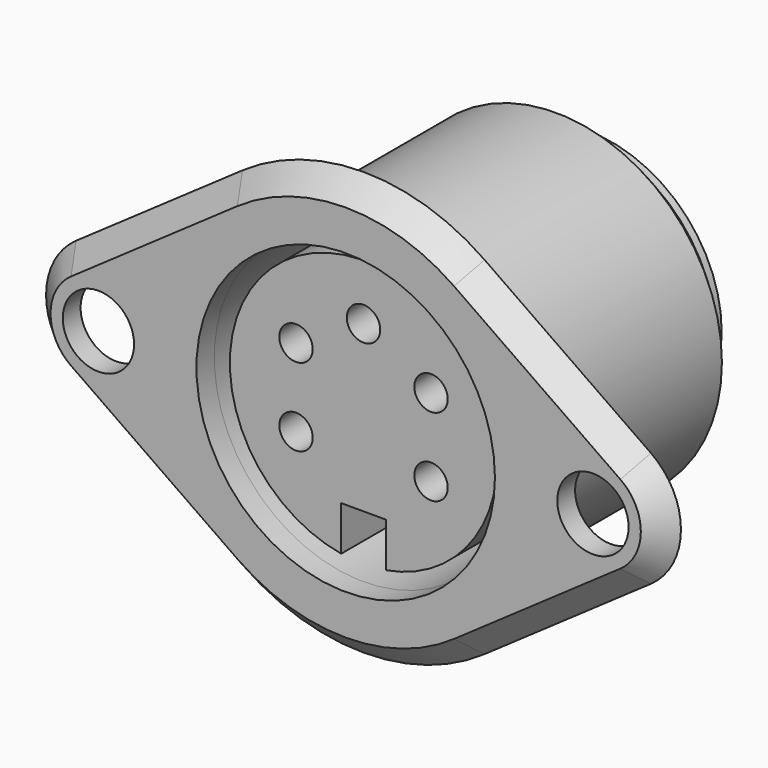
from build123d import *

# Parameters (mm, degrees)
F0_R     = 1.6
F0_R_2   = 7.45
F0_R_3   = 6.7
F1_DEPTH = 1
F2_SIZE  = 0.99999
F0_R_4   = 0.75
F3_DEPTH = 12.1
F4_T     = 0.75
F5_DEPTH = 12.6
F6_DEPTH = 10
F7_SIZE  = 1.3


# Not quite as in the source:
# - a fillet or chamfer is up to 0.001 mm smaller than in the source, because OpenCascade refuses the exact size
# - a shell that OpenCascade refuses in one call is made with other operations: the cavity is built on its own and cut out
# - a feature names something its author has since deleted; it is built from what else it names


with BuildPart() as f1:
    # F0 (on Front) → F1 (new body)
    with BuildSketch(Plane.XZ):
        with BuildLine():
            Line((-5.4346846847, 7.7919318771), (-12.902027027, 2.5836405698))
            ThreePointArc((-12.902027027, 2.5836405698), (-14.25, 0), (-12.902027027, -2.5836405698))
            Line((-12.902027027, -2.5836405698), (-5.4346846847, -7.7919318771))
            ThreePointArc((-5.4346846847, -7.7919318771), (0, -9.5), (5.4346846847, -7.7919318771))
            Line((5.4346846847, -7.7919318771), (12.902027027, -2.5836405698))
            ThreePointArc((12.902027027, -2.5836405698), (14.25, 0), (12.902027027, 2.5836405698))
            Line((12.902027027, 2.5836405698), (5.4346846847, 7.7919318771))
            ThreePointArc((5.4346846847, 7.7919318771), (0, 9.5), (-5.4346846847, 7.7919318771))
        make_face()
        with Locations((-11.1, 0)):
            Circle(F0_R, mode=Mode.SUBTRACT)
        Circle(F0_R_2, mode=Mode.SUBTRACT)
        with Locations((11.1, 0)):
            Circle(F0_R, mode=Mode.SUBTRACT)
        Circle(F0_R_2)
        Circle(F0_R_3, mode=Mode.SUBTRACT)
    extrude(amount=F1_DEPTH)

    # F2 (size 1 in the source; OpenCascade refuses exactly that, so slightly less here)
    f2_edges = [f1.edges().sort_by_distance(p)[0] for p in [
        (-9.168356, -1, 5.187786),
        (0, -1, 9.5),
        (-14.25, -1, 0),
        (-9.168356, -1, -5.187786),
        (0, -1, -9.5),
        (9.168356, -1, -5.187786),
        (14.25, -1, 0),
        (9.168356, -1, 5.187786),
    ]]
    chamfer(f2_edges, length=F2_SIZE)

    # F0 (on Front) → F3 (join)
    with BuildSketch(Plane.XZ):
        Circle(F0_R_2)
        Circle(F0_R_3, mode=Mode.SUBTRACT)
        Circle(F0_R_3)
        with BuildLine():
            ThreePointArc((-1, -5.9160797831), (-3.8729833462, 4.582575695), (6, 0))
            ThreePointArc((6, 0), (4.582575695, -3.8729833462), (1, -5.9160797831))
            Line((1, -5.9160797831), (1, -6.3300160691))
            Line((1, -6.3300160691), (-1, -6.3300160691))
            Line((-1, -6.3300160691), (-1, -5.9160797831))
        make_face(mode=Mode.SUBTRACT)
        with BuildLine():
            ThreePointArc((1, -5.9160797831), (4.582575695, -3.8729833462), (6, 0))
            ThreePointArc((6, 0), (-3.8729833462, 4.582575695), (-1, -5.9160797831))
            Line((-1, -5.9160797831), (-1, -3.9160797831))
            Line((-1, -3.9160797831), (0, -3.9160797831))
            Line((0, -3.9160797831), (1, -3.9160797831))
            Line((1, -3.9160797831), (1, -5.9160797831))
        make_face()
        with Locations((-3.0310889132, -1.75)):
            Circle(F0_R_4, mode=Mode.SUBTRACT)
        with Locations((3.0310889132, -1.75)):
            Circle(F0_R_4, mode=Mode.SUBTRACT)
        with Locations((-3.0310889132, 1.75)):
            Circle(F0_R_4, mode=Mode.SUBTRACT)
        with Locations((3.0310889132, 1.75)):
            Circle(F0_R_4, mode=Mode.SUBTRACT)
        with Locations((0, 3.5)):
            Circle(F0_R_4, mode=Mode.SUBTRACT)
        with Locations((-3.0310889132, -1.75)):
            Circle(F0_R_4)
        with BuildLine():
            Line((-1, -3.9160797831), (-1, -5.9160797831))
            ThreePointArc((-1, -5.9160797831), (0, -6), (1, -5.9160797831))
            Line((1, -5.9160797831), (1, -3.9160797831))
            Line((1, -3.9160797831), (0, -3.9160797831))
            Line((0, -3.9160797831), (-1, -3.9160797831))
        make_face()
        with BuildLine():
            ThreePointArc((1, -5.9160797831), (0, -6), (-1, -5.9160797831))
            Line((-1, -5.9160797831), (-1, -6.3300160691))
            Line((-1, -6.3300160691), (1, -6.3300160691))
            Line((1, -6.3300160691), (1, -5.9160797831))
        make_face()
        with Locations((-3.0310889132, 1.75)):
            Circle(F0_R_4)
        with Locations((0, 3.5)):
            Circle(F0_R_4)
        with Locations((3.0310889132, 1.75)):
            Circle(F0_R_4)
        with Locations((3.0310889132, -1.75)):
            Circle(F0_R_4)
    extrude(amount=-F3_DEPTH)

    # F4: shell of thickness 0.75, made by hand


with BuildPart() as f4_core1:
    # F4_t2: copy of F1
    add(f1.part)

    # the walls: a layer under each face that stays
    f4_faces = [f4_core1.faces().sort_by_distance(p)[0] for p in [
        (0, -5e-06, 9.5),
        (9.1683558559, -5e-06, 5.1877862235),
        (0, -0.500005, 9.000005),
        (-12.2142857143, 0, -2.7142857143),
        (-9.1683558559, -5e-06, 5.1877862235),
        (14.25, -5e-06, 0),
        (8.8823226802, -0.500005, 4.7776886467),
        (-8.83334, -1, 0),
        (-8.8823226802, -0.500005, 4.7776886467),
        (-14.25, -5e-06, 0),
        (9.1683558559, -5e-06, -5.1877862235),
        (-9.1683558559, -5e-06, -5.1877862235),
        (0, -5e-06, -9.5),
        (-12.7, -0.5, 0),
        (-7.45, 6.05, 0),
        (9.5, -0.5, 0),
        (13.750005, -0.500005, 0),
        (-13.750005, -0.500005, 0),
        (-8.8823226802, -0.500005, -4.7776886467),
        (0, -0.500005, -9.000005),
        (8.8823226802, -0.500005, -4.7776886467),
        (-6.7, -0.5, 0),
        (0, 12.1, 0),
    ]]
    thicken(f4_faces, amount=-F4_T, mode=Mode.SUBTRACT)

    # F4_s3 → F4_t4 (revolve, cut)
    with BuildSketch(Plane.XY):
        Polygon((7.4575, 0.0075), (7.45, -0.75), (6.7, -0.75), (6.7, 0), align=None)
    revolve(axis=Axis((0, 0, 0), (0, -1, 0)), mode=Mode.SUBTRACT)


with BuildPart() as f1_1:
    add(f1.part)

    # what is left inside the walls is the cavity
    f4_cavity = [f4_core1.part.solids().sort_by_distance(p)[0] for p in [
        (-6.6925, 7.566667, 0),
    ]]
    add(f4_cavity, mode=Mode.SUBTRACT)

    # F7
    f7_edges = [f1_1.edges().sort_by_distance(p)[0] for p in [
        (-7.45, 12.1, 0),
    ]]
    chamfer(f7_edges, length=F7_SIZE)


with BuildPart() as f5:
    # F0 (on Front) → F5 (new body)
    with BuildSketch(Plane.XZ):
        with BuildLine():
            ThreePointArc((1, -5.9160797831), (4.582575695, -3.8729833462), (6, 0))
            ThreePointArc((6, 0), (-3.8729833462, 4.582575695), (-1, -5.9160797831))
            Line((-1, -5.9160797831), (-1, -3.9160797831))
            Line((-1, -3.9160797831), (0, -3.9160797831))
            Line((0, -3.9160797831), (1, -3.9160797831))
            Line((1, -3.9160797831), (1, -5.9160797831))
        make_face()
        with Locations((-3.0310889132, -1.75)):
            Circle(F0_R_4, mode=Mode.SUBTRACT)
        with Locations((3.0310889132, -1.75)):
            Circle(F0_R_4, mode=Mode.SUBTRACT)
        with Locations((-3.0310889132, 1.75)):
            Circle(F0_R_4, mode=Mode.SUBTRACT)
        with Locations((3.0310889132, 1.75)):
            Circle(F0_R_4, mode=Mode.SUBTRACT)
        with Locations((0, 3.5)):
            Circle(F0_R_4, mode=Mode.SUBTRACT)
        with Locations((-3.0310889132, -1.75)):
            Circle(F0_R_4)
        with BuildLine():
            Line((-1, -3.9160797831), (-1, -5.9160797831))
            ThreePointArc((-1, -5.9160797831), (0, -6), (1, -5.9160797831))
            Line((1, -5.9160797831), (1, -3.9160797831))
            Line((1, -3.9160797831), (0, -3.9160797831))
            Line((0, -3.9160797831), (-1, -3.9160797831))
        make_face()
        with Locations((-3.0310889132, 1.75)):
            Circle(F0_R_4)
        with Locations((0, 3.5)):
            Circle(F0_R_4)
        with Locations((3.0310889132, 1.75)):
            Circle(F0_R_4)
        with Locations((3.0310889132, -1.75)):
            Circle(F0_R_4)
    extrude(amount=-F5_DEPTH)

    # F0 (on Front) → F6 (cut)
    with BuildSketch(Plane.XZ):
        with Locations((-3.0310889132, -1.75)):
            Circle(F0_R_4)
        with BuildLine():
            Line((-1, -3.9160797831), (-1, -5.9160797831))
            ThreePointArc((-1, -5.9160797831), (0, -6), (1, -5.9160797831))
            Line((1, -5.9160797831), (1, -3.9160797831))
            Line((1, -3.9160797831), (0, -3.9160797831))
            Line((0, -3.9160797831), (-1, -3.9160797831))
        make_face()
        with Locations((-3.0310889132, 1.75)):
            Circle(F0_R_4)
        with Locations((0, 3.5)):
            Circle(F0_R_4)
        with Locations((3.0310889132, 1.75)):
            Circle(F0_R_4)
        with Locations((3.0310889132, -1.75)):
            Circle(F0_R_4)
    extrude(amount=-F6_DEPTH, mode=Mode.SUBTRACT)


solid = Compound([f1_1.part, f5.part])
